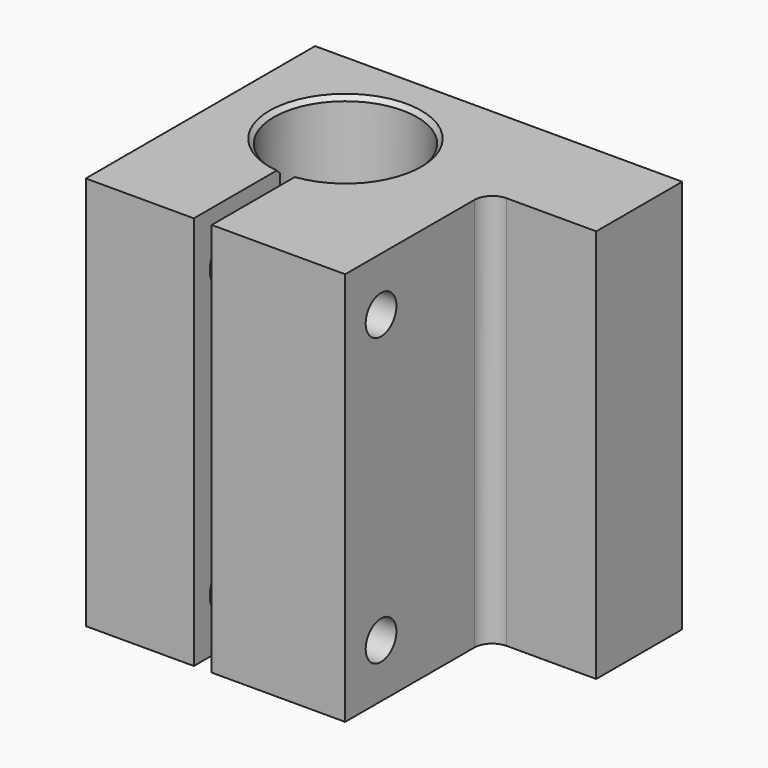
from build123d import *

# Parameters (mm, degrees)
F1_DEPTH       = 34.925
F3_D           = 8.8
F3_DEPTH       = 20.6375
F3_CBORE_D     = 14.25
F3_CBORE_DEPTH = 8
F3_TIP         = 2.6437867237
F5_D           = 6.8
F5_DEPTH       = 20.6375
F5_TIP         = 2.0429261047
F6_R           = 3.175
F7_SIZE        = 0.762
F9_D           = 6.8


# Not quite as in the source:
# - ends of sketch curves that miss each other by under 0.0002 mm in the source are joined


with BuildPart() as f1:
    # F0 (on Top) → F1 (new body, symmetric)
    with BuildSketch(Plane.XY):
        with BuildLine():
            Line((-30.1270424985, 1.5875), (-30.1270424985, -31.75))
            Line((-30.1270424985, -31.75), (-15.6690329313, -31.75))
            Line((-15.6690329313, -31.75), (-10.9754424985, -31.75))
            Line((-10.9754424985, -31.75), (-10.9754424985, -12.6142650107))
            ThreePointArc((-10.9754424985, -12.6142650107), (-19.4991930627, -7.8326866028), (-22.1026331175, 1.5875))
            ThreePointArc((-22.1026331175, 1.5875), (-0.5628331886, 9.0209179793), (-7.8004424985, -12.585462914))
            Line((-7.8004424985, -12.585462914), (-7.8004424985, -31.75))
            Line((-7.8004424985, -31.75), (15.8469575015, -31.75))
            Line((15.8469575015, -31.75), (15.8977575015, 0))
            Line((15.8977575015, 0), (34.9477575015, 0))
            Line((34.9477575015, 0), (34.9477575015, 19.05))
            Line((34.9477575015, 19.05), (-30.1270424985, 19.05))
            Line((-30.1270424985, 19.05), (-30.1270424985, 1.5875))
        make_face()
    extrude(amount=F1_DEPTH, both=True)

    # F3
    with Locations(Plane(origin=(-30.1270424985, 0, 0), x_dir=(0, -1, 0), z_dir=(-1, 0, 0))):
        with Locations((23.8125, 25.4), (23.8125, -25.4)):
            CounterBoreHole(F3_D / 2, F3_CBORE_D / 2, F3_CBORE_DEPTH, depth=F3_DEPTH)
            with Locations((0, 0, -(F3_DEPTH + F3_TIP / 2))):  # 118° drill point
                Cone(0, F3_D / 2, F3_TIP, mode=Mode.SUBTRACT)

    # F5
    with Locations(Plane(origin=(-30.1270424985, 0, 0), x_dir=(0, -1, 0), z_dir=(-1, 0, 0))):
        with Locations((24.2870002985, 0)):
            Hole(F5_D / 2, depth=F5_DEPTH)
            with Locations((0, 0, -(F5_DEPTH + F5_TIP / 2))):  # 118° drill point
                Cone(0, F5_D / 2, F5_TIP, mode=Mode.SUBTRACT)

    # F6
    f6_edges = [f1.edges().sort_by_distance(p)[0] for p in [
        (15.897758, 0, 0),
    ]]
    fillet(f6_edges, radius=F6_R)

    # F7
    f7_edges = [f1.edges().sort_by_distance(p)[0] for p in [
        (-9.617446, 12.699477, 34.925),
        (-9.617446, 12.699477, -34.925),
    ]]
    chamfer(f7_edges, length=F7_SIZE)

    # F9 (through all)
    with Locations(Plane(origin=(15.8977168033, -0.0254363469, 0), x_dir=(0.001599998, 0.99999872, 0), z_dir=(0.99999872, -0.001599998, 0))):
        with Locations((-23.7871042605, 25.4), (-23.7871042605, -25.4)):
            Hole(F9_D / 2)


solid = f1.part
